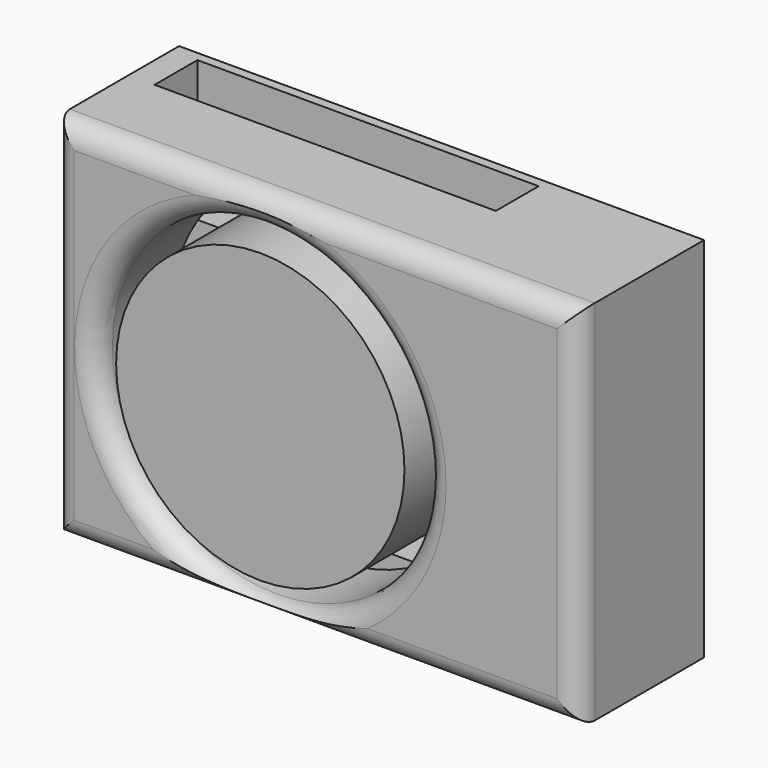
from build123d import *

# Parameters (mm, degrees)
F0_W         = 127
F0_H         = 88.9
F1_DEPTH     = 38.1
F2_W         = 127
F2_H         = 38.1
F2_W_2       = 82.55
F2_H_2       = 12.954
F3_DEPTH     = 25.4
F4_DEPTH     = 25.4
F5_W         = 44.1795827687
F5_H         = 12.954
F6_DEPTH     = 81.28
F7_R         = 39.8475218447
F7_R_2       = 34.8773795478
F8_DEPTH     = 22.86
F9_T3_DEPTH  = 152.4
F9_T6_DEPTH  = 114.3
F9_T9_DEPTH  = 114.3
F9_T12_DEPTH = 152.4


# Not quite as in the source:
# - a fillet or chamfer that OpenCascade refuses, or shapes differently, is made with other operations: its cross-section is extruded or revolved along the edge and cut away or added


with BuildPart() as f1:
    # F0 (on Front) → F1 (new body)
    with BuildSketch(Plane.XZ):
        with Locations((-63.5, -31.0818182497)):
            Rectangle(F0_W, F0_H)
    extrude(amount=F1_DEPTH)

    # F2 (on face) → F3 (join)
    with BuildSketch(Plane.XY.offset(13.3681817503)):
        with Locations((-63.5, -19.05)):
            Rectangle(F2_W, F2_H)
        with Locations((-79.4304944575, -8.7889100092)):
            Rectangle(F2_W_2, F2_H_2, mode=Mode.SUBTRACT)
    extrude(amount=-F3_DEPTH)

    # F2 (on face) → F4 (cut)
    with BuildSketch(Plane.XY.offset(13.3681817503)):
        with Locations((-79.4304944575, -8.7889100092)):
            Rectangle(F2_W_2, F2_H_2)
    extrude(amount=-F4_DEPTH, mode=Mode.SUBTRACT)

    # F5 (on face) → F6 (cut)
    with BuildSketch(Plane.XY.offset(13.3681817503)):
        with Locations((-60.2452858418, -8.7889100092)):
            Rectangle(F5_W, F5_H)
    extrude(amount=-F6_DEPTH, mode=Mode.SUBTRACT)

    # F7 (on face) → F8 (cut)
    with BuildSketch(Plane.XZ.offset(38.1)):
        with Locations((-76.8643096089, -33.7820015848)):
            Circle(F7_R)
        with Locations((-76.8643096089, -33.7820015848)):
            Circle(F7_R_2, mode=Mode.SUBTRACT)
    extrude(amount=-F8_DEPTH, mode=Mode.SUBTRACT)

    # F9: fillet of radius 5.08 on 5 edges, made by hand


with BuildPart() as f9_tool1:
    # F9_s2 → F9_t3 (new body)
    with BuildSketch(Plane.YZ.offset(12.7)):
        with BuildLine():
            ThreePointArc((-38.1, 8.2881817503), (-36.6121024484, 11.8802841987), (-33.02, 13.3681817503))
            Line((-33.02, 13.3681817503), (-38.1, 13.3681817503))
            Line((-38.1, 13.3681817503), (-38.1, 8.2881817503))
        make_face()
    extrude(amount=-F9_T3_DEPTH)


with BuildPart() as f9_tool4:
    # F9_s5 → F9_t6 (new body)
    with BuildSketch(Plane.XY.offset(-88.2318182497)):
        with BuildLine():
            ThreePointArc((-5.08, -38.1), (-1.4878975516, -36.6121024484), (0, -33.02))
            Line((0, -33.02), (0, -38.1))
            Line((0, -38.1), (-5.08, -38.1))
        make_face()
    extrude(amount=F9_T6_DEPTH)


with BuildPart() as f9_tool7:
    # F9_s8 → F9_t9 (new body)
    with BuildSketch(Plane.XY.offset(26.0681817503)):
        with BuildLine():
            ThreePointArc((-121.92, -38.1), (-125.5121024484, -36.6121024484), (-127, -33.02))
            Line((-127, -33.02), (-127, -38.1))
            Line((-127, -38.1), (-121.92, -38.1))
        make_face()
    extrude(amount=-F9_T9_DEPTH)


with BuildPart() as f9_tool10:
    # F9_s11 → F9_t12 (new body)
    with BuildSketch(Plane.YZ.offset(-139.7)):
        with BuildLine():
            ThreePointArc((-38.1, -70.4518182497), (-36.6121024484, -74.0439206982), (-33.02, -75.5318182497))
            Line((-33.02, -75.5318182497), (-38.1, -75.5318182497))
            Line((-38.1, -75.5318182497), (-38.1, -70.4518182497))
        make_face()
    extrude(amount=F9_T12_DEPTH)


with BuildPart() as f9_tool13:
    # F9_s14 → F9_t15 (revolve)
    with BuildSketch(Plane.XY.offset(-33.7820015848)):
        with BuildLine():
            ThreePointArc((-31.9367877642, -38.1), (-35.5288902127, -36.6121024484), (-37.0167877642, -33.02))
            Line((-37.0167877642, -33.02), (-37.0167877642, -38.1))
            Line((-37.0167877642, -38.1), (-31.9367877642, -38.1))
        make_face()
    revolve(axis=Axis((-76.8643096089, -38.1, -33.7820015848), (0, -1, 0)))


with BuildPart() as f1_1:
    add(f1.part)

    # F9_t16: cut F9_tool1, F9_tool4, F9_tool7, F9_tool10, F9_tool13
    add([f9_tool1.part, f9_tool4.part, f9_tool7.part, f9_tool10.part, f9_tool13.part], mode=Mode.SUBTRACT)


solid = f1_1.part
